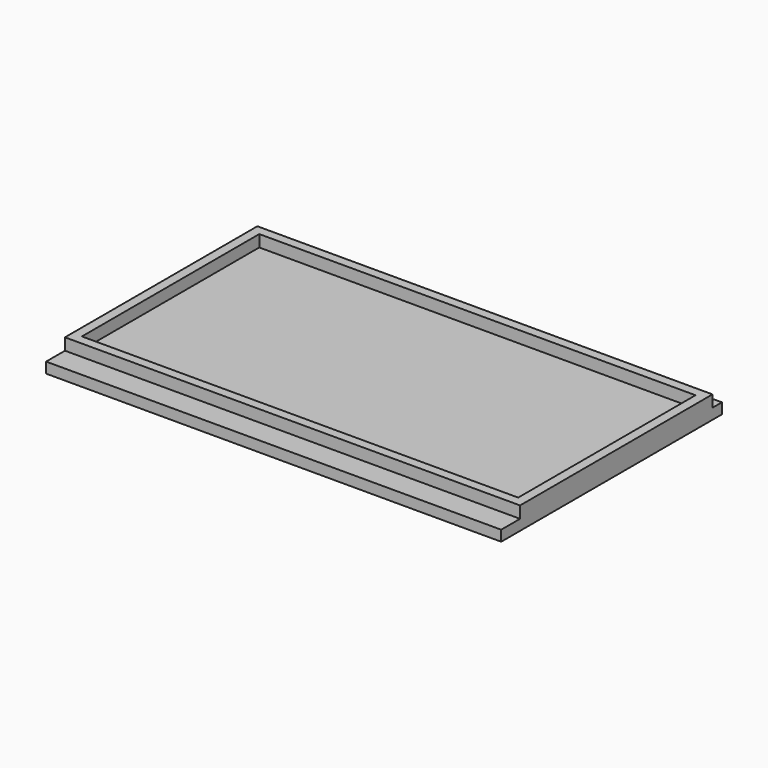
from build123d import *

# Parameters (mm, degrees)
F0_W     = 185
F0_H     = 94
F0_W_2   = 193
F0_H_2   = 10
F0_H_3   = 5
F1_DEPTH = 4.5
F2_DEPTH = 5


# Not quite as in the source:
# - a feature names something its author has since deleted; it is built from what else it names


with BuildPart() as f1:
    # F0 (on Top) → F1 (new body)
    with BuildSketch(Plane.XY):
        Polygon((96.5, 52), (96.5, 56), (-96.5, 56), (-96.5, 52), (-96.5, -42), (-96.5, -46), (96.5, -46), (96.5, -42), align=None)
        with Locations((0, 5)):
            Rectangle(F0_W, F0_H, mode=Mode.SUBTRACT)
        with Locations((0, 5)):
            Rectangle(F0_W, F0_H)
        with Locations((0, -51)):
            Rectangle(F0_W_2, F0_H_2)
        with Locations((0, 58.5)):
            Rectangle(F0_W_2, F0_H_3)
    extrude(amount=-F1_DEPTH)

    # F0 (on Top) → F2 (join)
    with BuildSketch(Plane.XY):
        Polygon((96.5, 52), (96.5, 56), (-96.5, 56), (-96.5, 52), (-96.5, -42), (-96.5, -46), (96.5, -46), (96.5, -42), align=None)
        with Locations((0, 5)):
            Rectangle(F0_W, F0_H, mode=Mode.SUBTRACT)
    extrude(amount=F2_DEPTH)


solid = f1.part
